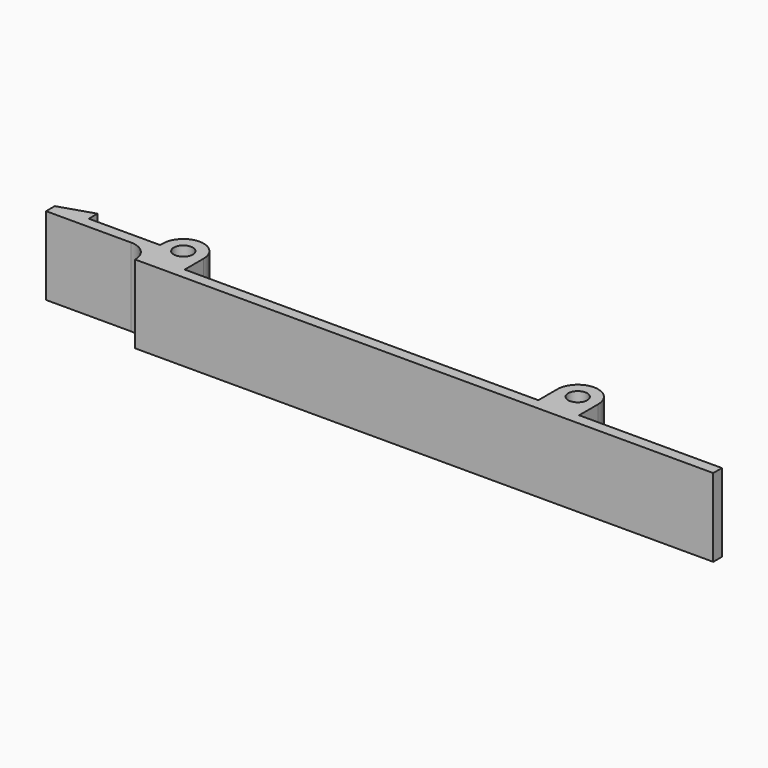
from build123d import *

# Parameters (mm, degrees)
F1_DEPTH = 11.5
F2_D     = 2.8
F3_R     = 2.99999


# Not quite as in the source:
# - a fillet or chamfer is up to 0.001 mm smaller than in the source, because OpenCascade refuses the exact size


with BuildPart() as f1:
    # F0 (on Top) → F1 (new body)
    with BuildSketch(Plane.XY):
        with BuildLine():
            Line((-61, -5.1), (24, -5.1))
            Line((24, -5.1), (24, -3.5))
            Line((24, -3.5), (3, -3.5))
            Line((3, -3.5), (3, 0))
            ThreePointArc((3, 0), (0, 3), (-3, 0))
            Line((-3, 0), (-3, -3.5))
            Line((-3, -3.5), (-55, -3.5))
            Line((-55, -3.5), (-55, 0))
            ThreePointArc((-55, 0), (-58, 3), (-61, 0))
            Line((-61, 0), (-61, -0.5))
            Line((-61, -0.5), (-71.5, -0.5))
            Line((-71.5, -0.5), (-71.5, 1.1))
            Line((-71.5, 1.1), (-76.5, -0.5))
            Line((-76.5, -0.5), (-76.5, -2.1))
            Line((-76.5, -2.1), (-61, -2.1))
            Line((-61, -2.1), (-61, -5.1))
        make_face()
    extrude(amount=F1_DEPTH)

    # F2 (through all)
    with Locations(Plane(origin=(0, 0, 0), x_dir=(1, 0, 0), z_dir=(0, 0, -1))):
        with Locations((-58, 0), (0, 0)):
            Hole(F2_D / 2)

    # F3 (radius 3 in the source; OpenCascade refuses exactly that, so slightly less here)
    f3_edges = [f1.edges().sort_by_distance(p)[0] for p in [
        (-61, -2.1, 5.75),
    ]]
    fillet(f3_edges, radius=F3_R)


solid = f1.part
